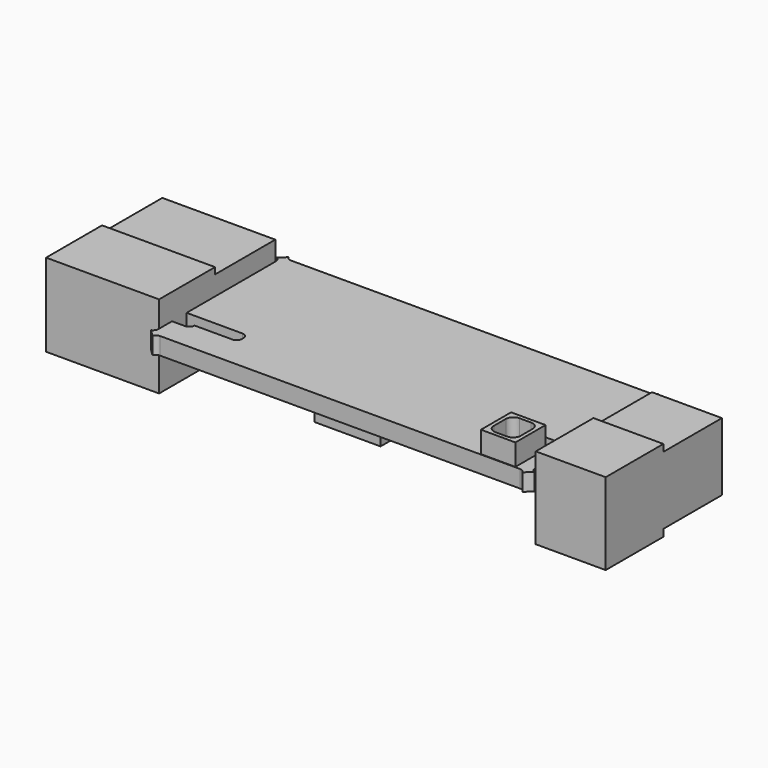
from build123d import *

# Parameters (mm, degrees)
F1_DEPTH  = 1.6
F3_DEPTH  = 10.5
F5_START  = 35
F5_DEPTH  = 6.5
F6_W      = 3.2
F6_H      = 3.5
F7_DEPTH  = 3.6
F8_W      = 3
F8_H      = 4.3
F9_DEPTH  = 4.5
F10_W     = 5.15
F10_H     = 6.15
F10_W_2   = 6.15
F10_H_2   = 5.15
F11_DEPTH = 1.1


with BuildPart() as f1:
    # F0 (on Top) → F1 (new body)
    with BuildSketch(Plane.XY):
        with BuildLine():
            Line((1.2, 15.2), (0.7727922061, 15.2))
            ThreePointArc((0.7727922061, 15.2), (0.4943088368, 15.2847326006), (0.3102119479, 15.5102119479))
            Line((0.3102119479, 15.5102119479), (-0.3102119479, 14.8897880521))
            ThreePointArc((-0.3102119479, 14.8897880521), (-0.0847326006, 14.7056911632), (0, 14.4272077939))
            Line((0, 14.4272077939), (0, 4.05))
            Line((0, 4.05), (5.2, 4.05))
            ThreePointArc((5.2, 4.05), (5.5535533906, 3.9035533906), (5.7, 3.55))
            Line((5.7, 3.55), (5.7, 3.35))
            ThreePointArc((5.7, 3.35), (5.5535533906, 2.9964466094), (5.2, 2.85))
            Line((5.2, 2.85), (1.7, 2.85))
            ThreePointArc((1.7, 2.85), (1.5535533906, 2.4964466094), (1.2, 2.35))
            Line((1.2, 2.35), (0, 2.35))
            Line((0, 2.35), (0, 0.7727922061))
            ThreePointArc((0, 0.7727922061), (-0.0847326006, 0.4943088368), (-0.3102119479, 0.3102119479))
            Line((-0.3102119479, 0.3102119479), (0.3102119479, -0.3102119479))
            ThreePointArc((0.3102119479, -0.3102119479), (0.4943088368, -0.0847326006), (0.7727922061, 0))
            Line((0.7727922061, 0), (1.2, 0))
            Line((1.2, 0), (33.8, 0))
            Line((33.8, 0), (34.2272077939, 0))
            ThreePointArc((34.2272077939, 0), (34.5056911632, -0.0847326006), (34.6897880521, -0.3102119479))
            Line((34.6897880521, -0.3102119479), (35.3102119479, 0.3102119479))
            ThreePointArc((35.3102119479, 0.3102119479), (35.0847326006, 0.4943088368), (35, 0.7727922061))
            Line((35, 0.7727922061), (35, 3.85))
            Line((35, 3.85), (30, 3.85))
            ThreePointArc((30, 3.85), (29.6464466094, 3.9964466094), (29.5, 4.35))
            Line((29.5, 4.35), (29.5, 4.55))
            ThreePointArc((29.5, 4.55), (29.6464466094, 4.9035533906), (30, 5.05))
            Line((30, 5.05), (35, 5.05))
            Line((35, 5.05), (35, 14.4272077939))
            ThreePointArc((35, 14.4272077939), (35.0847326006, 14.7056911632), (35.3102119479, 14.8897880521))
            Line((35.3102119479, 14.8897880521), (34.6897880521, 15.5102119479))
            ThreePointArc((34.6897880521, 15.5102119479), (34.5056911632, 15.2847326006), (34.2272077939, 15.2))
            Line((34.2272077939, 15.2), (33.8, 15.2))
            Line((33.8, 15.2), (1.2, 15.2))
        make_face()
    extrude(amount=F1_DEPTH)

    # F2 (on Right) → F3 (join)
    with BuildSketch(Plane.YZ):
        Polygon((7.35, 4), (0.85, 4), (0.85, -3.7), (7.35, -3.7), (7.35, -3.1), (14.35, -3.1), (14.35, 3.4), (7.35, 3.4), align=None)
    extrude(amount=-F3_DEPTH)

    # F4 (on Right) → F5 (join)
    with BuildSketch(Plane.YZ.offset(F5_START)):
        Polygon((7.55, 2.95), (0.85, 2.95), (0.85, -4.65), (7.55, -4.65), (7.55, -4), (14.35, -4), (14.35, 2.3), (7.55, 2.3), align=None)
    extrude(amount=F5_DEPTH)

    # F6 (on Top) → F7 (join)
    with BuildSketch(Plane.XY):
        with Locations((32.15, 1.8)):
            Rectangle(F6_W, F6_H)
        with BuildLine():
            ThreePointArc((30.9, 2.5), (31.1050252532, 2.9949747468), (31.6, 3.2))
            Line((31.6, 3.2), (32.7, 3.2))
            ThreePointArc((32.7, 3.2), (33.1949747468, 2.9949747468), (33.4, 2.5))
            Line((33.4, 2.5), (33.4, 1.1))
            ThreePointArc((33.4, 1.1), (33.1949747468, 0.6050252532), (32.7, 0.4))
            Line((32.7, 0.4), (31.6, 0.4))
            ThreePointArc((31.6, 0.4), (31.1050252532, 0.6050252532), (30.9, 1.1))
            Line((30.9, 1.1), (30.9, 2.5))
        make_face(mode=Mode.SUBTRACT)
    extrude(amount=F7_DEPTH)

    # F8 (on Top) → F9 (join)
    with BuildSketch(Plane.XY):
        with Locations((25.5, 12.95)):
            Rectangle(F8_W, F8_H)
    extrude(amount=-F9_DEPTH)

    # F10 (on Top) → F11 (join)
    with BuildSketch(Plane.XY):
        with Locations((10.9508251641, 9.2315472887)):
            Rectangle(F10_W, F10_H)
        with Locations((16.9374256049, 10.8333893863)):
            Rectangle(F10_W, F10_H)
        with Locations((17.7855274571, 3.0699999196)):
            Rectangle(F10_W_2, F10_H_2)
    extrude(amount=-F11_DEPTH)


solid = f1.part
